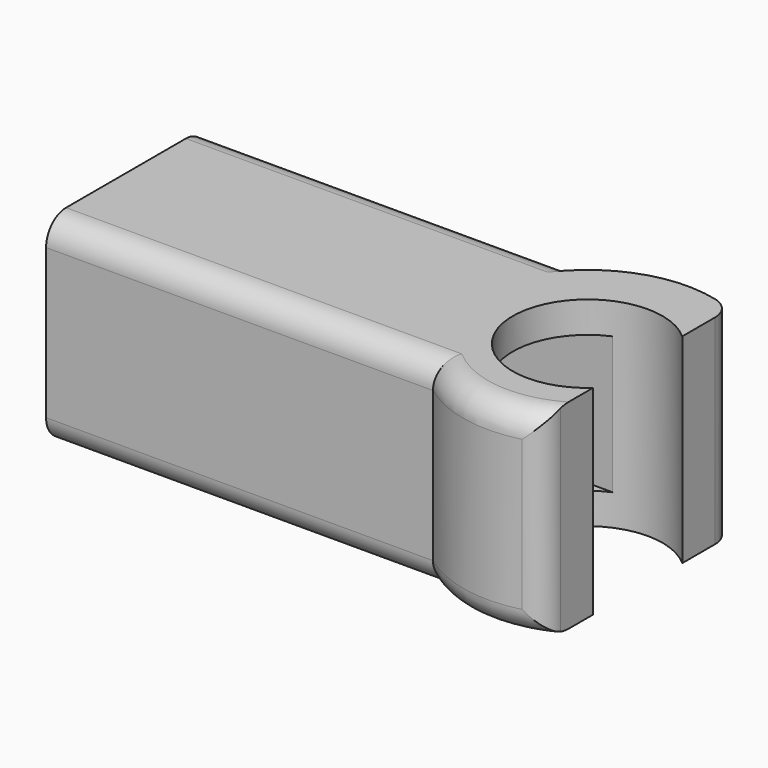
from build123d import *

# Parameters (mm, degrees)
F1_DEPTH = 8
F2_W     = 5.5
F2_H     = 5.5
F3_DEPTH = 17.3020421192
F4_R     = 1


# Not quite as in the source:
# - a feature names something its author has since deleted; it is built from what else it names


with BuildPart() as f1:
    # F0 (on Top) → F1 (new body)
    with BuildSketch(Plane.XY):
        with BuildLine():
            ThreePointArc((2, -2.2360679775), (-3, 0), (2, 2.2360679775))
            Line((2, 2.2360679775), (2, 4.582575695))
            ThreePointArc((2, 4.582575695), (-0.5786610494, 4.9664022582), (-3, 4))
            ThreePointArc((-3, 4), (-5, 0), (-3, -4))
            ThreePointArc((-3, -4), (-0.5786610494, -4.9664022582), (2, -4.582575695))
            Line((2, -4.582575695), (2, -2.2360679775))
        make_face()
        with BuildLine():
            ThreePointArc((-3, -4), (-5, 0), (-3, 4))
            Line((-3, 4), (-18.5, 4))
            Line((-18.5, 4), (-18.5, -4))
            Line((-18.5, -4), (-3, -4))
        make_face()
    extrude(amount=F1_DEPTH)

    # F2 (on face) → F3 (cut, through all)
    with BuildSketch(Plane(origin=(-18.5, 0, 0), x_dir=(0, -1, 0), z_dir=(-1, 0, 0))):
        with Locations((0, 4)):
            Rectangle(F2_W, F2_H)
    extrude(amount=-F3_DEPTH, mode=Mode.SUBTRACT)

    # F4
    f4_edges = [f1.edges().sort_by_distance(p)[0] for p in [
        (2, 4.582576, 4),
        (2, -4.582576, 4),
        (-10.75, -4, 0),
        (-10.75, 4, 8),
        (-10.75, 4, 0),
        (-10.75, -4, 8),
        (-0.578661, -4.966402, 8),
        (-0.578661, -4.966402, 0),
    ]]
    fillet(f4_edges, radius=F4_R)


solid = f1.part
